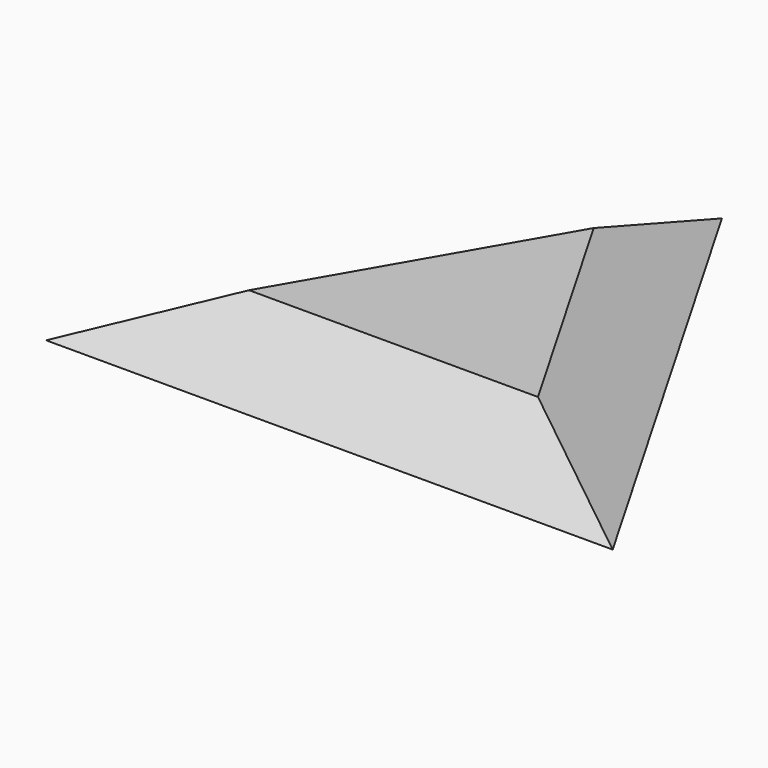
from build123d import *

# Parameters (mm, degrees)
F1_DEPTH = 5
F2_SIZE2 = 7.072207
F2_SIZE  = 4.99999


# Not quite as in the source:
# - a fillet or chamfer is up to 0.001 mm smaller than in the source, because OpenCascade refuses the exact size


with BuildPart() as f1:
    # F0 (on Top) → F1 (new body)
    with BuildSketch(Plane.XY):
        Polygon((0, 28.8675134595), (-25, -14.4337567297), (25, -14.4337567297), align=None)
    extrude(amount=F1_DEPTH)

    # F2 (size 5 and 7.0722171527 in the source; OpenCascade refuses exactly that, so slightly less here)
    f2_edges = [f1.edges().sort_by_distance(p)[0] for p in [
        (-12.5, 7.216878, 5),
        (12.5, 7.216878, 5),
        (0, -14.433757, 5),
    ]]
    chamfer(f2_edges, length=F2_SIZE, length2=F2_SIZE2)


solid = f1.part
